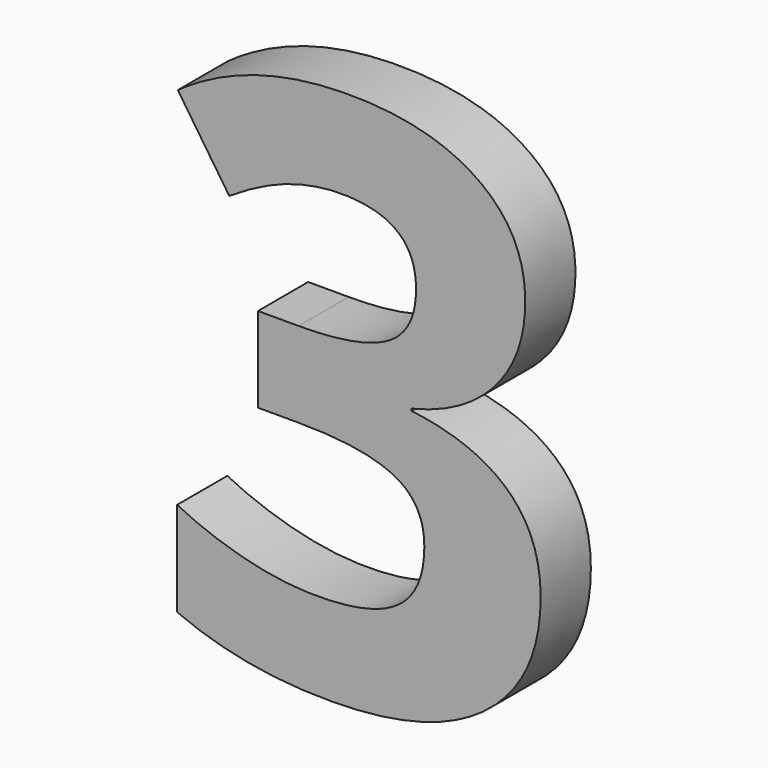
from build123d import *

# Parameters (mm, degrees)
F0_TEXT_SIZE = 74.4517038889
F1_DEPTH     = 6.35


# Not quite as in the source:
# - Text() gives the source's letters only with a copy of the font that has no kerning and outlines rounded to 1/6400 em; it was checked with that copy


with BuildPart() as f1:
    # F0 (on Front) → F1 (new body)
    with BuildSketch(Plane.XZ):
        with Locations((-44.6300377657, -16.1061568709)):
            Text('3', F0_TEXT_SIZE, font='Open Sans', font_style=FontStyle.BOLD, text_align=(TextAlign.LEFT, TextAlign.BOTTOM))
    extrude(amount=F1_DEPTH)


solid = f1.part
